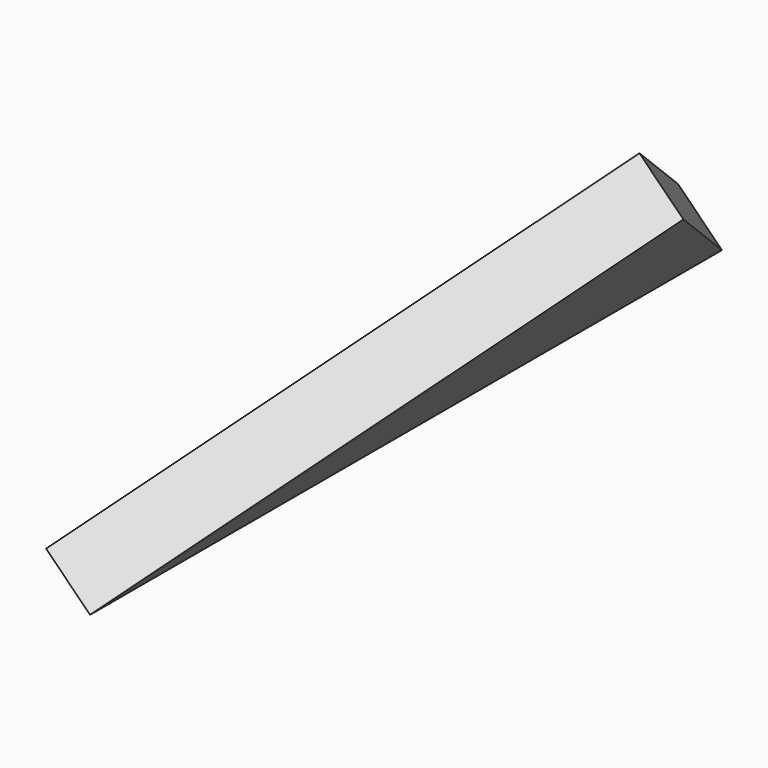
from build123d import *

# Parameters (mm, degrees)
F2_DEPTH = 2
F3_ANGLE = 45


# Not quite as in the source:
# - a feature of the source that left no trace in its solid (it failed there, or was rolled back) is left out


with BuildPart() as f2:
    # F0 (on Top) → F2 (new body)
    with BuildSketch(Plane.XY):
        Polygon((0, 0), (-12.7356738907, 12.8062811768), (-12.7356738907, -12.5937188232), align=None)
    extrude(amount=F2_DEPTH)


with BuildPart() as f2_1:
    # F3: moved
    add(f2.part.rotate(Axis((-12.7356738907, 0.1062811768, 0), (0, -1, 0)), F3_ANGLE))


solid = f2_1.part
